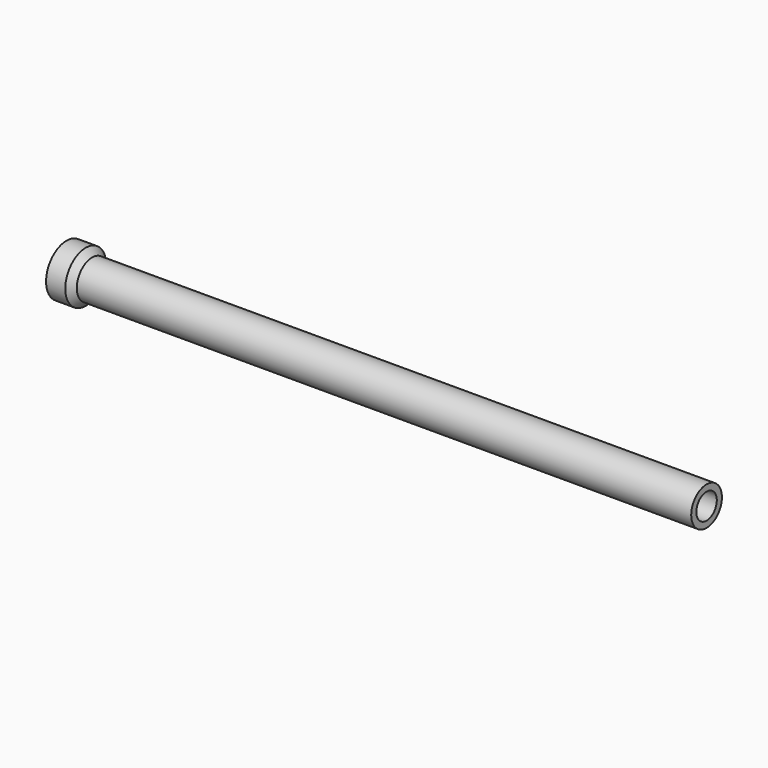
from build123d import *

# Parameters (mm, degrees)
F2_SIZE = 25.39999


# Not quite as in the source:
# - a fillet or chamfer is up to 0.001 mm smaller than in the source, because OpenCascade refuses the exact size


with BuildPart() as f1:
    # F0 (on Front) → F1 (revolve)
    with BuildSketch(Plane.XZ):
        Polygon((-1219.2, 50.8), (1270, 50.8), (1270, 76.2), (-1168.4, 76.2), (-1168.4, 101.6), (-1219.2, 101.6), (-1270, 101.6), (-1270, 76.2), (-1219.2, 76.2), align=None)
    revolve(axis=Axis((0, 0, 0), (-1, 0, 0)))

    # F2 (size 25.4 in the source; OpenCascade refuses exactly that, so slightly less here)
    f2_edges = [f1.edges().sort_by_distance(p)[0] for p in [
        (-1168.4, 0, -101.6),
    ]]
    chamfer(f2_edges, length=F2_SIZE)


solid = f1.part
